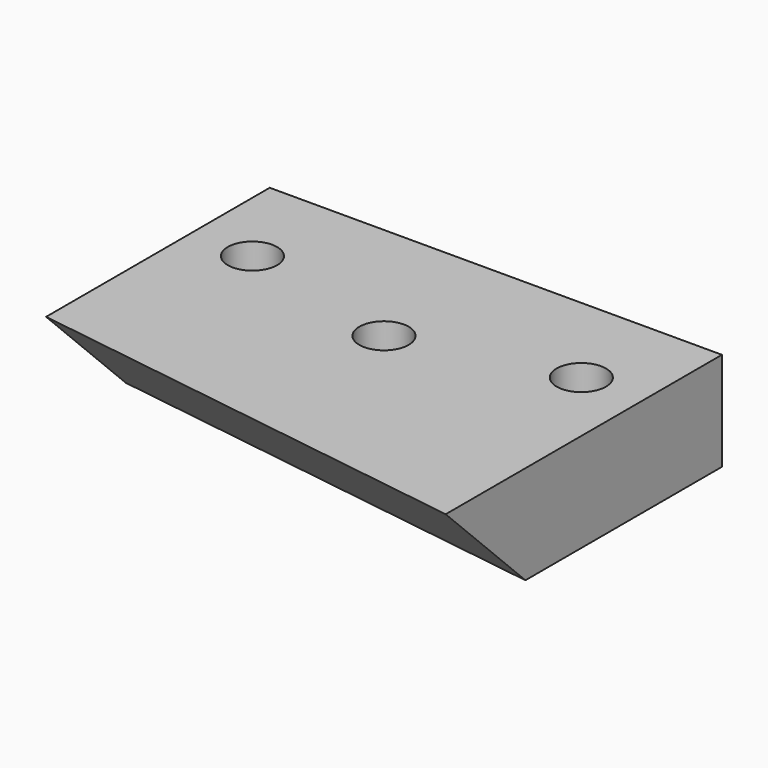
from build123d import *

# Parameters (mm, degrees)
F1_DEPTH = 6
F2_SIZE  = 5.99999
F3_R     = 1.5
F4_DEPTH = 6


# Not quite as in the source:
# - a fillet or chamfer is up to 0.001 mm smaller than in the source, because OpenCascade refuses the exact size


with BuildPart() as f1:
    # F0 (on Top) → F1 (new body)
    with BuildSketch(Plane.XY):
        Polygon((23.7662842423, 6.9127185345), (-3.7337157577, 6.9127185345), (-3.7337157577, -10.0872814655), (23.7662842423, -14.0872814655), align=None)
    extrude(amount=F1_DEPTH)

    # F2 (size 6 in the source; OpenCascade refuses exactly that, so slightly less here)
    f2_edges = [f1.edges().sort_by_distance(p)[0] for p in [
        (10.016284, -12.087281, 0),
    ]]
    chamfer(f2_edges, length=F2_SIZE)

    # F3 (on face) → F4 (cut, through all)
    with BuildSketch(Plane.XY.offset(6)):
        with Locations((0.0162842423, 0.9127185345)):
            Circle(F3_R)
        with Locations((10.0162842423, -1.5872814655)):
            Circle(F3_R)
        with Locations((20.0162842423, 0.9127185345)):
            Circle(F3_R)
    extrude(amount=-F4_DEPTH, mode=Mode.SUBTRACT)


solid = f1.part
